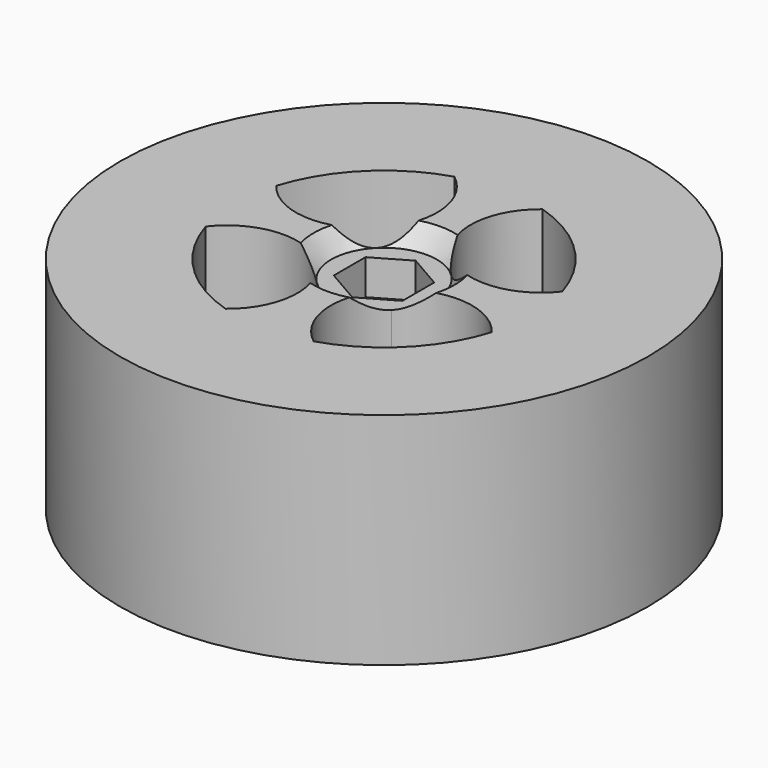
from build123d import *

# Parameters (mm, degrees)
F0_R     = 30
F0_R_2   = 3
F1_DEPTH = 25
F2_START = 2
F0_R_3   = 2.75
F2_DEPTH = 21
F4_DEPTH = 6
F5_START = 19
F5_DEPTH = 4


# Not quite as in the source:
# - a fillet or chamfer that OpenCascade refuses, or shapes differently, is made with other operations: its cross-section is extruded or revolved along the edge and cut away or added
# - a feature names something its author has since deleted; it is built from what else it names


with BuildPart() as f1:
    # F0 (on Top) → F1 (new body)
    with BuildSketch(Plane.XY):
        Circle(F0_R)
        with BuildLine():
            ThreePointArc((16.2480768093, 5), (16.8109682314, 2.5281113744), (17, 0))
            ThreePointArc((17, 0), (16.8109682314, -2.5281113744), (16.2480768093, -5))
            ThreePointArc((16.2480768093, -5), (12.0208152802, -12.0208152802), (5, -16.2480768093))
            ThreePointArc((5, -16.2480768093), (0, -17), (-5, -16.2480768093))
            ThreePointArc((-5, -16.2480768093), (-12.0208152802, -12.0208152802), (-16.2480768093, -5))
            ThreePointArc((-16.2480768093, -5), (-17, 0), (-16.2480768093, 5))
            ThreePointArc((-16.2480768093, 5), (-12.0208152802, 12.0208152802), (-5, 16.2480768093))
            ThreePointArc((-5, 16.2480768093), (0, 17), (5, 16.2480768093))
            ThreePointArc((5, 16.2480768093), (12.0208152802, 12.0208152802), (16.2480768093, 5))
        make_face(mode=Mode.SUBTRACT)
        with BuildLine():
            ThreePointArc((16.2480768093, -5), (16.8109682314, -2.5281113744), (17, 0))
            ThreePointArc((17, 0), (16.8109682314, 2.5281113744), (16.2480768093, 5))
            ThreePointArc((16.2480768093, 5), (10.4163777832, 1.9103772572), (4.2426406998, 4.2426406745))
            ThreePointArc((4.2426406998, 4.2426406745), (5.5432771985, 2.2961005859), (6, 0))
            ThreePointArc((6, 0), (5.5432771928, -2.2961005997), (4.2426406787, -4.2426406956))
            ThreePointArc((4.2426406787, -4.2426406956), (10.4163777683, -1.9103772563), (16.2480768093, -5))
        make_face()
        with BuildLine():
            ThreePointArc((4.2426406998, 4.2426406745), (1.9103772561, 10.4163777654), (5, 16.2480768093))
            ThreePointArc((5, 16.2480768093), (0, 17), (-5, 16.2480768093))
            ThreePointArc((-5, 16.2480768093), (-1.9103772567, 10.4163777743), (-4.2426406871, 4.2426406871))
            ThreePointArc((-4.2426406871, 4.2426406871), (8.9e-09, 6), (4.2426406998, 4.2426406745))
        make_face()
        with BuildLine():
            ThreePointArc((6, 0), (5.5432771985, 2.2961005859), (4.2426406998, 4.2426406745))
            ThreePointArc((4.2426406998, 4.2426406745), (8.9e-09, 6), (-4.2426406871, 4.2426406871))
            ThreePointArc((-4.2426406871, 4.2426406871), (-6, 4e-10), (-4.2426406877, -4.2426406865))
            ThreePointArc((-4.2426406877, -4.2426406865), (-6.4e-09, -6), (4.2426406787, -4.2426406956))
            ThreePointArc((4.2426406787, -4.2426406956), (5.5432771928, -2.2961005997), (6, 0))
        make_face()
        Polygon((0, -4.5033320997), (-3.9, -2.2516660498), (-3.9, 2.2516660498), (0, 4.5033320997), (3.9, 2.2516660498), (3.9, -2.2516660498), align=None, mode=Mode.SUBTRACT)
        with BuildLine():
            ThreePointArc((-5, -16.2480768093), (0, -17), (5, -16.2480768093))
            ThreePointArc((5, -16.2480768093), (1.910377257, -10.4163777803), (4.2426406787, -4.2426406956))
            ThreePointArc((4.2426406787, -4.2426406956), (-6.4e-09, -6), (-4.2426406877, -4.2426406865))
            ThreePointArc((-4.2426406877, -4.2426406865), (-1.9103772566, -10.4163777739), (-5, -16.2480768093))
        make_face()
        with BuildLine():
            ThreePointArc((-4.2426406877, -4.2426406865), (-6, 4e-10), (-4.2426406871, 4.2426406871))
            ThreePointArc((-4.2426406871, 4.2426406871), (-10.4163777743, 1.9103772567), (-16.2480768093, 5))
            ThreePointArc((-16.2480768093, 5), (-17, 0), (-16.2480768093, -5))
            ThreePointArc((-16.2480768093, -5), (-10.4163777747, -1.9103772567), (-4.2426406877, -4.2426406865))
        make_face()
        Polygon((-3.9, 2.2516660498), (-3.9, -2.2516660498), (0, -4.5033320997), (3.9, -2.2516660498), (3.9, 2.2516660498), (0, 4.5033320997), align=None)
        Circle(F0_R_2, mode=Mode.SUBTRACT)
    extrude(amount=F1_DEPTH)

    # F0 (on Top) → F2 (join)
    with BuildSketch(Plane.XY.offset(F2_START)):
        Circle(F0_R_2)
        Circle(F0_R_3, mode=Mode.SUBTRACT)
    extrude(amount=F2_DEPTH)

    # F3: chamfer of 5 on 2 edges, made by hand


with BuildPart() as f3_tool2:
    # F3_s3 → F3_t4 (revolve)
    with BuildSketch(Plane.XZ):
        Polygon((8, 0), (3, 5), (3, 0), align=None)
    revolve(axis=Axis((0, 0, 0), (0, 0, 1)))

    split(bisect_by=Plane.XY.offset(2), keep=Keep.BOTTOM)


with BuildPart() as f1_1:
    add(f1.part)

    # F3_t1: cut F3_tool2
    add(f3_tool2.part, mode=Mode.SUBTRACT)


with BuildPart() as f3_tool7:
    # F3_s8 → F3_t9 (revolve)
    with BuildSketch(Plane.XZ):
        Polygon((8, 25), (3, 20), (3, 25), align=None)
    revolve(axis=Axis((0, 0, 25), (0, 0, 1)))

    split(bisect_by=Plane.XY.offset(23), keep=Keep.TOP)


with BuildPart() as f1_2:
    add(f1_1.part)

    # F3_t6: cut F3_tool7
    add(f3_tool7.part, mode=Mode.SUBTRACT)

    # F0 (on Top) → F4 (cut)
    with BuildSketch(Plane.XY):
        Polygon((-3.9, 2.2516660498), (-3.9, -2.2516660498), (0, -4.5033320997), (3.9, -2.2516660498), (3.9, 2.2516660498), (0, 4.5033320997), align=None)
        Circle(F0_R_2, mode=Mode.SUBTRACT)
        Circle(F0_R_2)
        Circle(F0_R_3, mode=Mode.SUBTRACT)
        Circle(F0_R_3)
    extrude(amount=F4_DEPTH, mode=Mode.SUBTRACT)

    # F0 (on Top) → F5 (cut)
    with BuildSketch(Plane.XY.offset(F5_START)):
        Polygon((-3.9, 2.2516660498), (-3.9, -2.2516660498), (0, -4.5033320997), (3.9, -2.2516660498), (3.9, 2.2516660498), (0, 4.5033320997), align=None)
        Circle(F0_R_2, mode=Mode.SUBTRACT)
        Circle(F0_R_2)
        Circle(F0_R_3, mode=Mode.SUBTRACT)
    extrude(amount=F5_DEPTH, mode=Mode.SUBTRACT)


solid = f1_2.part
